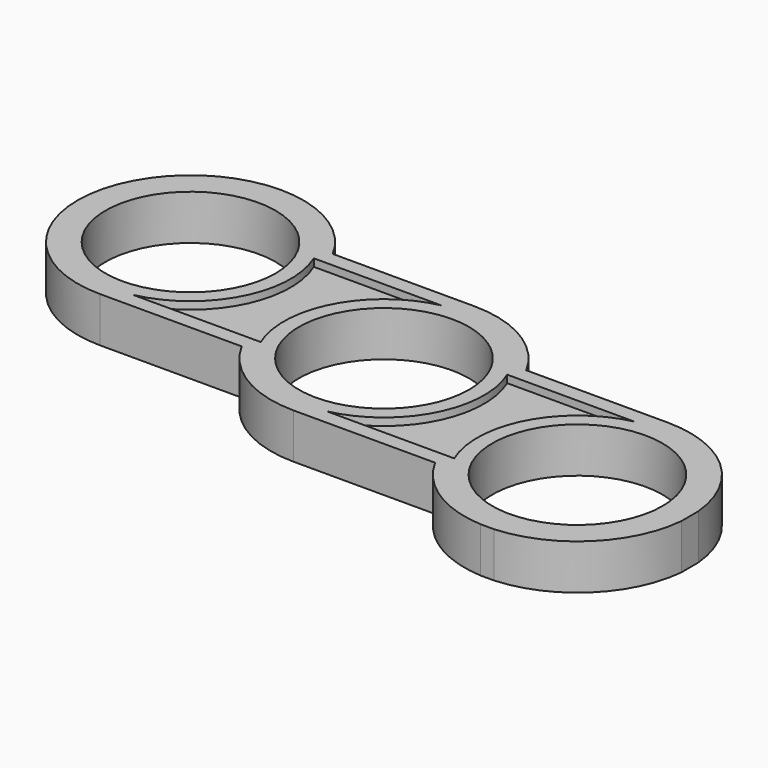
from build123d import *

# Parameters (mm, degrees)
F0_R        = 14.351
F1_DEPTH    = 7.62
F2_T        = 2.54
F2_T3_DEPTH = 12.7
F4_DEPTH    = 7.62
F5_DEPTH    = 1.27
F7_DEPTH    = 1.27


# Not quite as in the source:
# - a shell that OpenCascade refuses in one call is made with other operations: the cavity is built on its own and cut out


with BuildPart() as f1:
    # F0 (on Top) → F1 (new body)
    with BuildSketch(Plane.XY):
        with BuildLine():
            ThreePointArc((-40.64, -9.05), (-27.1696158184, -3.4703841816), (-21.59, 10))
            ThreePointArc((-21.59, 10), (-22.1705835176, 14.6672427406), (-23.8769453858, 19.05))
            ThreePointArc((-23.8769453858, 19.05), (-30.880389352, 26.3600886306), (-40.64, 29.05))
            ThreePointArc((-40.64, 29.05), (-54.0574684375, 23.5230928684), (-59.6894143559, 10.1493743547))
            ThreePointArc((-59.6894143559, 10.1493743547), (-54.1630928684, -3.4174684375), (-40.64, -9.05))
        make_face()
        with Locations((-40.64, 10)):
            Circle(F0_R, mode=Mode.SUBTRACT)
        with BuildLine():
            ThreePointArc((-23.8769453858, 19.05), (-22.1705835176, 14.6672427406), (-21.59, 10))
            ThreePointArc((-21.59, 10), (-27.1696158184, -3.4703841816), (-40.64, -9.05))
            Line((-40.64, -9.05), (-16.7630546142, -9.05))
            ThreePointArc((-16.7630546142, -9.05), (-16.3600886306, 9.759610648), (0, 19.05))
            Line((0, 19.05), (-23.8769453858, 19.05))
        make_face()
        with BuildLine():
            ThreePointArc((16.7630546142, 9.05), (9.759610648, 16.3600886306), (0, 19.05))
            ThreePointArc((0, 19.05), (-16.3600886306, 9.759610648), (-16.7630546142, -9.05))
            ThreePointArc((-16.7630546142, -9.05), (-9.759610648, -16.3600886306), (0, -19.05))
            ThreePointArc((0, -19.05), (13.4703841816, -13.4703841816), (19.05, 0))
            ThreePointArc((19.05, 0), (18.4694164824, 4.6672427406), (16.7630546142, 9.05))
        make_face()
        Circle(F0_R, mode=Mode.SUBTRACT)
        with BuildLine():
            Line((40.64, 9.05), (16.7630546142, 9.05))
            ThreePointArc((16.7630546142, 9.05), (18.4694164824, 4.6672427406), (19.05, 0))
            ThreePointArc((19.05, 0), (13.4703841816, -13.4703841816), (0, -19.05))
            Line((0, -19.05), (23.8769453858, -19.05))
            ThreePointArc((23.8769453858, -19.05), (24.2799113694, -0.240389352), (40.64, 9.05))
        make_face()
        with BuildLine():
            ThreePointArc((59.6056254338, -8.2090360401), (53.4615567808, 4.0893641346), (40.64, 9.05))
            ThreePointArc((40.64, 9.05), (24.2799113694, -0.240389352), (23.8769453858, -19.05))
            ThreePointArc((23.8769453858, -19.05), (30.3891760199, -26.0568710442), (39.4861384834, -29.0150231028))
            Line((39.4861384834, -29.0150231028), (41.7938615166, -29.0150231028))
            ThreePointArc((41.7938615166, -29.0150231028), (53.8825636539, -23.6944152074), (59.6056254338, -11.7909639599))
            Line((59.6056254338, -11.7909639599), (59.6056254338, -8.2090360401))
        make_face()
        with Locations((40.64, -10)):
            Circle(F0_R, mode=Mode.SUBTRACT)
    extrude(amount=F1_DEPTH)

    # F2: shell of thickness 2.54, made by hand


with BuildPart() as f2_core1:
    # F2_t2: copy of F1
    add(f1.part)

    # the walls: a layer under each face that stays
    f2_faces = [f2_core1.faces().sort_by_distance(p)[0] for p in [
        (-57.0000886306, 19.759610648, 3.81),
        (-28.7015273071, -9.05, 3.81),
        (-9.759610648, -16.3600886306, 3.81),
        (11.9384726929, -19.05, 3.81),
        (30.3891760199, -26.0568710442, 3.81),
        (40.64, -29.0150231028, 3.81),
        (53.8825636539, -23.6944152074, 3.81),
        (59.6056254338, -10, 3.81),
        (53.4615567808, 4.0893641346, 3.81),
        (28.7015273071, 9.05, 3.81),
        (9.759610648, 16.3600886306, 3.81),
        (-11.9384726929, 19.05, 3.81),
        (-54.991, 10, 3.81),
        (-14.351, 0, 3.81),
        (26.289, -10, 3.81),
        (-51.1688838976, 0.0174884486, 0),
    ]]
    thicken(f2_faces, amount=-F2_T, mode=Mode.SUBTRACT)

    # F2_s4 → F2_t3 (cut)
    with BuildSketch(Plane.XY.offset(-2.54)):
        Polygon((-23.8545946463, 19.0874666667), (-26.1120193343, 17.8433333333), (-25.3921823509, 16.51), (-23.8769453858, 16.51), align=None)
        Polygon((-16.7854053537, -9.0874666667), (-16.7630546142, -6.51), (-15.2478176491, -6.51), (-14.5279806657, -7.8433333333), align=None)
        Polygon((23.8545946463, -19.0874666667), (23.8769453858, -16.51), (25.3921823509, -16.51), (26.1120193343, -17.8433333333), align=None)
        Polygon((16.7854053537, 9.0874666667), (16.7630546142, 6.51), (15.2478176491, 6.51), (14.5279806657, 7.8433333333), align=None)
    extrude(amount=F2_T3_DEPTH, mode=Mode.SUBTRACT)


with BuildPart() as f1_1:
    add(f1.part)

    # what is left inside the walls is the cavity
    f2_cavity = [f2_core1.part.solids().sort_by_distance(p)[0] for p in [
        (-20.32, 1.163333, 7.5946),
        (20.32, -8.836667, 7.5946),
    ]]
    add(f2_cavity, mode=Mode.SUBTRACT)

    # F3 (on face) → F4 (join)
    with BuildSketch(Plane.XY.offset(7.62)):
        with BuildLine():
            ThreePointArc((-15.5860765108, -6.51), (-14.9730845713, 7.8174560709), (-3.5673212639, 16.51))
            Line((-3.5673212639, 16.51), (-25.0539234892, 16.51))
            ThreePointArc((-25.0539234892, 16.51), (-25.6669154287, 2.1825439291), (-37.0726787361, -6.51))
            Line((-37.0726787361, -6.51), (-15.5860765108, -6.51))
        make_face()
        with BuildLine():
            ThreePointArc((25.0539234892, -16.51), (25.6669154287, -2.1825439291), (37.0726787361, 6.51))
            Line((37.0726787361, 6.51), (15.5860765108, 6.51))
            ThreePointArc((15.5860765108, 6.51), (14.9730845713, -7.8174560709), (3.5673212639, -16.51))
            Line((3.5673212639, -16.51), (25.0539234892, -16.51))
        make_face()
    extrude(amount=-F4_DEPTH)

    # F3 (on face) → F5 (cut)
    with BuildSketch(Plane.XY.offset(7.62)):
        with BuildLine():
            ThreePointArc((-15.5860765108, -6.51), (-14.9730845713, 7.8174560709), (-3.5673212639, 16.51))
            Line((-3.5673212639, 16.51), (-25.0539234892, 16.51))
            ThreePointArc((-25.0539234892, 16.51), (-25.6669154287, 2.1825439291), (-37.0726787361, -6.51))
            Line((-37.0726787361, -6.51), (-15.5860765108, -6.51))
        make_face()
        with BuildLine():
            ThreePointArc((25.0539234892, -16.51), (25.6669154287, -2.1825439291), (37.0726787361, 6.51))
            Line((37.0726787361, 6.51), (15.5860765108, 6.51))
            ThreePointArc((15.5860765108, 6.51), (14.9730845713, -7.8174560709), (3.5673212639, -16.51))
            Line((3.5673212639, -16.51), (25.0539234892, -16.51))
        make_face()
    extrude(amount=-F5_DEPTH, mode=Mode.SUBTRACT)

    # F6 (on face) → F7 (cut)
    with BuildSketch(Plane(origin=(0, 0, 0), x_dir=(1, 0, 0), z_dir=(0, 0, -1))):
        with BuildLine():
            Line((-15.5860765108, 6.51), (-37.0726787361, 6.51))
            ThreePointArc((-37.0726787361, 6.51), (-25.6669154287, -2.1825439291), (-25.0539234892, -16.51))
            Line((-25.0539234892, -16.51), (-3.5673212639, -16.51))
            ThreePointArc((-3.5673212639, -16.51), (-14.9730845713, -7.8174560709), (-15.5860765108, 6.51))
        make_face()
        with BuildLine():
            Line((15.5860765108, -6.51), (37.0726787361, -6.51))
            ThreePointArc((37.0726787361, -6.51), (25.6669154287, 2.1825439291), (25.0539234892, 16.51))
            Line((25.0539234892, 16.51), (3.5673212639, 16.51))
            ThreePointArc((3.5673212639, 16.51), (14.9730845713, 7.8174560709), (15.5860765108, -6.51))
        make_face()
    extrude(amount=-F7_DEPTH, mode=Mode.SUBTRACT)


solid = f1_1.part
